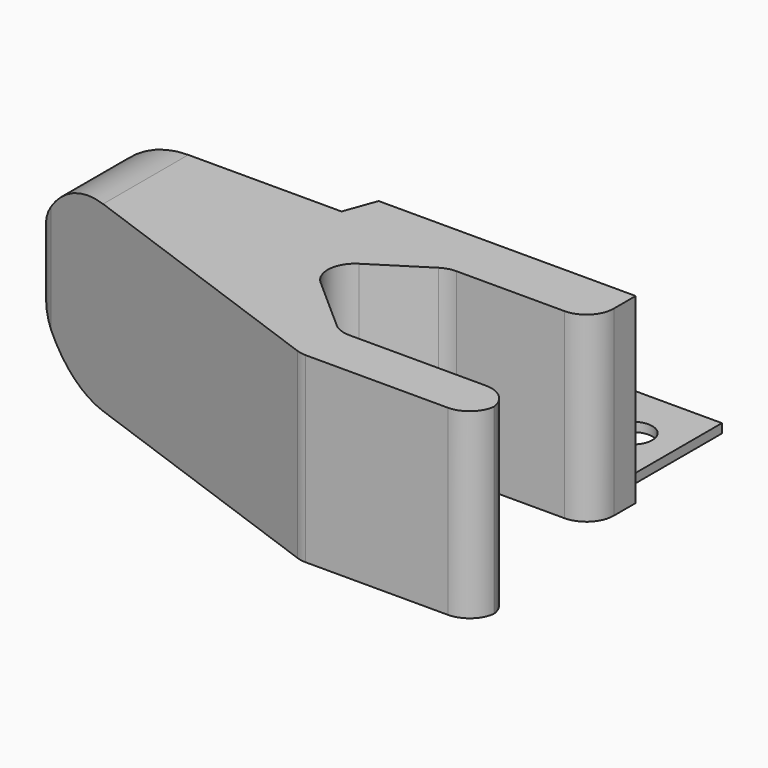
from build123d import *

# Parameters (mm, degrees)
F0_R      = 10
F0_R_2    = 6.25
F0_R_3    = 1.5
F1_DEPTH  = 1.5
F2_SIZE   = 1.49999
F3_R      = 10
F3_R_2    = 6.25
F4_DEPTH  = 2
F5_R      = 2
F6_W      = 12.5
F6_H      = 2.2
F7_DEPTH  = 10
F8_R      = 2.1
F9_DEPTH  = 5
F11_DEPTH = 22.7357939163
F10_R     = 6.25
F12_DEPTH = 2.2
F13_R     = 1.5
F13_W     = 24.693130475
F13_H     = 12.4008059502
F13_R_2   = 2.1
F14_DEPTH = 1
F15_ANGLE = -90


# Not quite as in the source:
# - a fillet or chamfer is up to 0.001 mm smaller than in the source, because OpenCascade refuses the exact size


with BuildPart() as f1:
    # F0 (on Top) → F1 (new body)
    with BuildSketch(Plane.XY):
        with Locations((-15, 0)):
            Circle(F0_R)
        with Locations((-15, 0)):
            Circle(F0_R_2, mode=Mode.SUBTRACT)
        with Locations((-15, 0)):
            Circle(F0_R_2)
        with Locations((-15, 0)):
            Circle(F0_R_3, mode=Mode.SUBTRACT)
    extrude(amount=F1_DEPTH)

    # F2 (size 1.5 in the source; OpenCascade refuses exactly that, so slightly less here)
    f2_edges = [f1.edges().sort_by_distance(p)[0] for p in [
        (-16.5, 0, 1.5),
    ]]
    chamfer(f2_edges, length=F2_SIZE)

    # F3 (on face) → F4 (join)
    with BuildSketch(Plane.XY.offset(1.5)):
        with Locations((-15, 0)):
            Circle(F3_R)
        with Locations((-15, 0)):
            Circle(F3_R_2, mode=Mode.SUBTRACT)
    extrude(amount=F4_DEPTH)

    # F5
    f5_edges = [f1.edges().sort_by_distance(p)[0] for p in [
        (-25, 0, 3.5),
    ]]
    fillet(f5_edges, radius=F5_R)


with BuildPart() as f7:
    # F6 (on Front) → F7 (new body, symmetric)
    with BuildSketch(Plane.XZ):
        with BuildLine():
            Line((-25, 3.5), (-23, 3.5))
            Line((-23, 3.5), (-21.25, 3.5))
            Line((-21.25, 3.5), (-21.25, 5.7))
            Line((-21.25, 5.7), (-8.75, 5.7))
            Line((-8.75, 5.7), (-8.75, 3.5))
            Line((-8.75, 3.5), (-7, 3.5))
            Line((-7, 3.5), (1.8147304989, 3.5))
            Line((1.8147304989, 3.5), (3.082514781, 0))
            Line((3.082514781, 0), (31.2739014626, 0))
            Line((31.2739014626, 0), (31.2739014626, 3))
            ThreePointArc((31.2739014626, 3), (30.3952218061, 5.1213203436), (28.2739014626, 6))
            Line((28.2739014626, 6), (16.4085253357, 6))
            ThreePointArc((16.4085253357, 6), (15.5703347425, 6.119472873), (14.7989048414, 6.4683756471))
            Line((14.7989048414, 6.4683756471), (9.028848419, 10.1370088155))
            ThreePointArc((9.028848419, 10.1370088155), (7.6477576678, 12.4327386036), (8.6518544799, 14.9166018275))
            Line((8.6518544799, 14.9166018275), (14.684603133, 20.2479686592))
            ThreePointArc((14.684603133, 20.2479686592), (15.6091219911, 20.8057000889), (16.6712175665, 21))
            Line((16.6712175665, 21), (31.6612296999, 21))
            ThreePointArc((31.6612296999, 21), (33.6426674196, 21.7474670784), (34.6367321637, 23.6173969582))
            ThreePointArc((34.6367321637, 23.6173969582), (33.6426674196, 25.4873268379), (31.6612296999, 26.2347939163))
            Line((31.6612296999, 26.2347939163), (16.0621650929, 26.2347939163))
            ThreePointArc((16.0621650929, 26.2347939163), (15.5434996934, 26.1896181418), (15.0404550345, 26.0554513852))
            Line((15.0404550345, 26.0554513852), (-23.0217100584, 12.2684186281))
            ThreePointArc((-23.0217100584, 12.2684186281), (-24.4561280682, 11.170385585), (-25, 9.4477611592))
            Line((-25, 9.4477611592), (-25, 3.5))
        make_face()
        with Locations((-15, 4.6)):
            Rectangle(F6_W, F6_H)
    extrude(amount=F7_DEPTH, both=True)

    # F8 (on face) → F9 (cut)
    with BuildSketch(Plane(origin=(0, 0, 0), x_dir=(1, 0, 0), z_dir=(0, 0, -1))):
        with Locations((12, 0)):
            Circle(F8_R)
        with Locations((23, 0)):
            Circle(F8_R)
    extrude(amount=-F9_DEPTH, mode=Mode.SUBTRACT)

    # F10 (on face) → F11 (cut, through all)
    with BuildSketch(Plane(origin=(0, 0, 3.5), x_dir=(1, 0, 0), z_dir=(0, 0, -1))):
        with BuildLine():
            ThreePointArc((-25, 0), (-22.0710678119, 7.0710678119), (-15, 10))
            Line((-15, 10), (-25, 10))
            Line((-25, 10), (-25, 0))
        make_face()
        with BuildLine():
            Line((-25, -10), (-15, -10))
            ThreePointArc((-15, -10), (-22.0710678119, -7.0710678119), (-25, 0))
            Line((-25, 0), (-25, -10))
        make_face()
    extrude(amount=-F11_DEPTH, mode=Mode.SUBTRACT)

    # F10 (on face) → F12 (cut)
    with BuildSketch(Plane(origin=(0, 0, 3.5), x_dir=(1, 0, 0), z_dir=(0, 0, -1))):
        with Locations((-15, 0)):
            Circle(F10_R)
    extrude(amount=-F12_DEPTH, mode=Mode.SUBTRACT)


with BuildPart() as f14:
    # F13 (on face) → F14 (new body)
    with BuildSketch(Plane(origin=(0, 0, 0), x_dir=(1, 0, 0), z_dir=(0, 0, -1))):
        Polygon((3.082514781, 6.2004029751), (0, 6.2004029751), (0, 3.361225361), (-19.286269322, 3.361225361), (-19.286269322, -3.361225361), (0, -3.361225361), (0, -6.2004029751), (3.082514781, -6.2004029751), align=None)
        with Locations((-15, 0)):
            Circle(F13_R, mode=Mode.SUBTRACT)
        with Locations((15.4290800185, 0)):
            Rectangle(F13_W, F13_H)
        with Locations((12, 0)):
            Circle(F13_R_2, mode=Mode.SUBTRACT)
        with Locations((23, 0)):
            Circle(F13_R_2, mode=Mode.SUBTRACT)
    extrude(amount=F14_DEPTH)


with BuildPart() as f7_1:
    # F15: moved
    add(f7.part.rotate(Axis((17.1782081218, -10, 0), (-1, 0, 0)), F15_ANGLE))


solid = Compound([f1.part, f14.part, f7_1.part])
